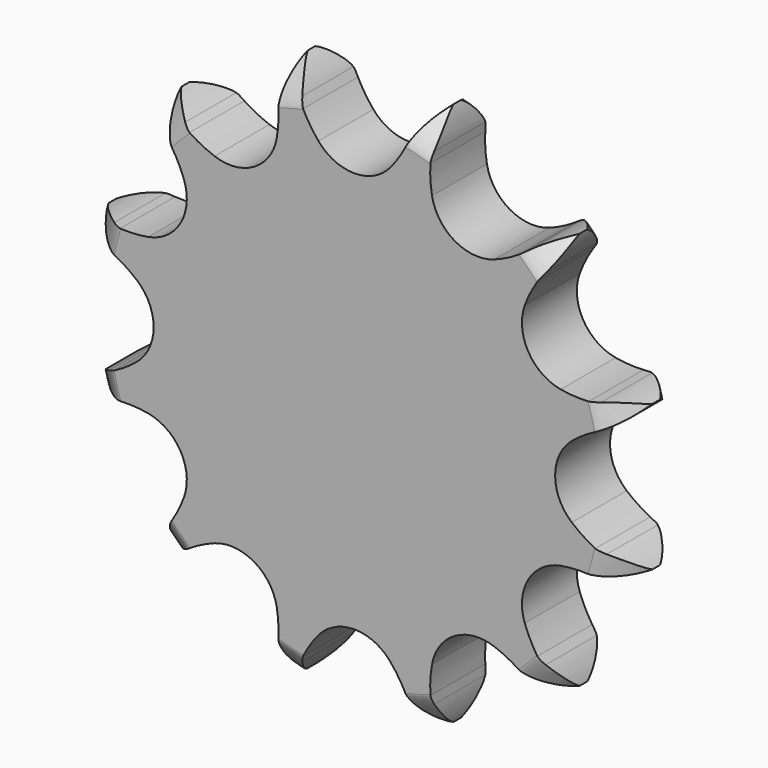
from build123d import *

# Parameters (mm, degrees)
F5_DEPTH = 5.1013001


# Not quite as in the source:
# - a fillet or chamfer that OpenCascade refuses, or shapes differently, is made with other operations: its cross-section is extruded or revolved along the edge and cut away or added


with BuildPart() as f1:
    # F0 (on Right) → F1 (revolve)
    with BuildSketch(Plane.YZ):
        Polygon((5.1003, 21), (0, 21), (0, 0), (5.1003, 0), (5.1003, 15), align=None)
    revolve(axis=Axis((0, 2.55015, 0), (0, 1, 0)))

    # F2: fillet of radius 2.75 on 1 edges, made by hand

    # F2_s1 → F2_t2 (revolve, cut)
    with BuildSketch(Plane.YZ):
        with BuildLine():
            add(Edge.make_bspline(
                [(2.75, 21), (0, 21), (0, 18.25)],
                knots=[0, 0, 0, 1, 1, 1], degree=2, weights=[1, 0.25, 1]))
            Line((0, 18.25), (0, 21))
            Line((0, 21), (2.75, 21))
        make_face()
    revolve(axis=Axis((0, 0, 0), (0, 1, 0)), mode=Mode.SUBTRACT)

    # F3: fillet of radius 2.25 on 1 edges, made by hand

    # F3_s1 → F3_t2 (revolve, cut)
    with BuildSketch(Plane.YZ):
        with BuildLine():
            add(Edge.make_bspline(
                [(2.8503, 21), (5.1003, 21), (5.1003, 18.75)],
                knots=[0, 0, 0, 1, 1, 1], degree=2, weights=[1, 0.25, 1]))
            Line((5.1003, 18.75), (5.1003, 21))
            Line((5.1003, 21), (2.8503, 21))
        make_face()
    revolve(axis=Axis((0, 5.1003, 0), (0, 1, 0)), mode=Mode.SUBTRACT)

    # F4 (on Front) → F5 (intersect, through all)
    with BuildSketch(Plane.XZ):
        with BuildLine():
            ThreePointArc((2.6688988398, 16.1610279679), (0, 14.9165), (-2.6688988398, 16.1610279679))
            ThreePointArc((-2.6688988398, 16.1610279679), (-3.2918405608, 16.997783911), (-3.8134287394, 17.9012011279))
            Line((-3.8134287394, 17.9012011279), (-4.1168666624, 18.5053956993))
            ThreePointArc((-4.1168666624, 18.5053956993), (-4.6860108551, 19.4160194738), (-5.4140261854, 20.2054207974))
            ThreePointArc((-5.4140261854, 20.2054207974), (-5.6498052939, 19.1577715323), (-5.6873867361, 18.0845761139))
            Line((-5.6873867361, 18.0845761139), (-5.6480744001, 17.4096093047))
            ThreePointArc((-5.6480744001, 17.4096093047), (-5.6480744046, 16.3664329553), (-5.7691797885, 15.3303101913))
            ThreePointArc((-5.7691797885, 15.3303101913), (-7.45825, 12.9180679356), (-10.3918481793, 12.6614113515))
            ThreePointArc((-10.3918481793, 12.6614113515), (-11.3497095063, 13.0745923945), (-12.2531267278, 13.5961805653))
            Line((-12.2531267278, 13.5961805653), (-12.8180089633, 13.9677094515))
            ThreePointArc((-12.8180089633, 13.9677094515), (-13.7662141799, 14.4717606771), (-14.791394612, 14.791394612))
            ThreePointArc((-14.791394612, 14.791394612), (-14.4717606771, 13.7662141799), (-13.9677094515, 12.8180089633))
            Line((-13.9677094515, 12.8180089633), (-13.5961805653, 12.2531267278))
            ThreePointArc((-13.5961805653, 12.2531267278), (-13.0745923945, 11.3497095063), (-12.6614113515, 10.3918481793))
            ThreePointArc((-12.6614113515, 10.3918481793), (-12.9180679356, 7.45825), (-15.3303101913, 5.7691797885))
            ThreePointArc((-15.3303101913, 5.7691797885), (-16.3664329553, 5.6480744046), (-17.4096093047, 5.6480744001))
            Line((-17.4096093047, 5.6480744001), (-18.0845761139, 5.6873867361))
            ThreePointArc((-18.0845761139, 5.6873867361), (-19.1577715323, 5.6498052939), (-20.2054207974, 5.4140261854))
            ThreePointArc((-20.2054207974, 5.4140261854), (-19.4160194738, 4.6860108551), (-18.5053956993, 4.1168666624))
            Line((-18.5053956993, 4.1168666624), (-17.9012011279, 3.8134287394))
            ThreePointArc((-17.9012011279, 3.8134287394), (-16.997783911, 3.2918405608), (-16.1610279679, 2.6688988398))
            ThreePointArc((-16.1610279679, 2.6688988398), (-14.9165, 0), (-16.1610279679, -2.6688988398))
            ThreePointArc((-16.1610279679, -2.6688988398), (-16.997783911, -3.2918405608), (-17.9012011279, -3.8134287394))
            Line((-17.9012011279, -3.8134287394), (-18.5053956993, -4.1168666624))
            ThreePointArc((-18.5053956993, -4.1168666624), (-19.4160194738, -4.6860108551), (-20.2054207974, -5.4140261854))
            ThreePointArc((-20.2054207974, -5.4140261854), (-19.1577715323, -5.6498052939), (-18.0845761139, -5.6873867361))
            Line((-18.0845761139, -5.6873867361), (-17.4096093047, -5.6480744001))
            ThreePointArc((-17.4096093047, -5.6480744001), (-16.3664329553, -5.6480744046), (-15.3303101913, -5.7691797885))
            ThreePointArc((-15.3303101913, -5.7691797885), (-12.9180679356, -7.45825), (-12.6614113515, -10.3918481793))
            ThreePointArc((-12.6614113515, -10.3918481793), (-13.0745923945, -11.3497095063), (-13.5961805653, -12.2531267278))
            Line((-13.5961805653, -12.2531267278), (-13.9677094515, -12.8180089633))
            ThreePointArc((-13.9677094515, -12.8180089633), (-14.4717606771, -13.7662141799), (-14.791394612, -14.791394612))
            ThreePointArc((-14.791394612, -14.791394612), (-13.7662141799, -14.4717606771), (-12.8180089633, -13.9677094515))
            Line((-12.8180089633, -13.9677094515), (-12.2531267278, -13.5961805653))
            ThreePointArc((-12.2531267278, -13.5961805653), (-11.3497095063, -13.0745923945), (-10.3918481793, -12.6614113515))
            ThreePointArc((-10.3918481793, -12.6614113515), (-7.45825, -12.9180679356), (-5.7691797885, -15.3303101913))
            ThreePointArc((-5.7691797885, -15.3303101913), (-5.6480744046, -16.3664329553), (-5.6480744001, -17.4096093047))
            Line((-5.6480744001, -17.4096093047), (-5.6873867361, -18.0845761139))
            ThreePointArc((-5.6873867361, -18.0845761139), (-5.6498052939, -19.1577715323), (-5.4140261854, -20.2054207974))
            ThreePointArc((-5.4140261854, -20.2054207974), (-4.6860108551, -19.4160194738), (-4.1168666624, -18.5053956993))
            Line((-4.1168666624, -18.5053956993), (-3.8134287394, -17.9012011279))
            ThreePointArc((-3.8134287394, -17.9012011279), (-3.2918405608, -16.997783911), (-2.6688988398, -16.1610279679))
            ThreePointArc((-2.6688988398, -16.1610279679), (0, -14.9165), (2.6688988398, -16.1610279679))
            ThreePointArc((2.6688988398, -16.1610279679), (3.2918405608, -16.997783911), (3.8134287394, -17.9012011279))
            Line((3.8134287394, -17.9012011279), (4.1168666624, -18.5053956993))
            ThreePointArc((4.1168666624, -18.5053956993), (4.6860108551, -19.4160194738), (5.4140261854, -20.2054207974))
            ThreePointArc((5.4140261854, -20.2054207974), (5.6498052939, -19.1577715323), (5.6873867361, -18.0845761139))
            Line((5.6873867361, -18.0845761139), (5.6480744001, -17.4096093047))
            ThreePointArc((5.6480744001, -17.4096093047), (5.6480744046, -16.3664329553), (5.7691797885, -15.3303101913))
            ThreePointArc((5.7691797885, -15.3303101913), (7.45825, -12.9180679356), (10.3918481793, -12.6614113515))
            ThreePointArc((10.3918481793, -12.6614113515), (11.3497095063, -13.0745923945), (12.2531267278, -13.5961805653))
            Line((12.2531267278, -13.5961805653), (12.8180089633, -13.9677094515))
            ThreePointArc((12.8180089633, -13.9677094515), (13.7662141799, -14.4717606771), (14.791394612, -14.791394612))
            ThreePointArc((14.791394612, -14.791394612), (14.4717606771, -13.7662141799), (13.9677094515, -12.8180089633))
            Line((13.9677094515, -12.8180089633), (13.5961805653, -12.2531267278))
            ThreePointArc((13.5961805653, -12.2531267278), (13.0745923945, -11.3497095063), (12.6614113515, -10.3918481793))
            ThreePointArc((12.6614113515, -10.3918481793), (12.9180679356, -7.45825), (15.3303101913, -5.7691797885))
            ThreePointArc((15.3303101913, -5.7691797885), (16.3664329553, -5.6480744046), (17.4096093047, -5.6480744001))
            Line((17.4096093047, -5.6480744001), (18.0845761139, -5.6873867361))
            ThreePointArc((18.0845761139, -5.6873867361), (19.1577715323, -5.6498052939), (20.2054207974, -5.4140261854))
            ThreePointArc((20.2054207974, -5.4140261854), (19.4160194738, -4.6860108551), (18.5053956993, -4.1168666624))
            Line((18.5053956993, -4.1168666624), (17.9012011279, -3.8134287394))
            ThreePointArc((17.9012011279, -3.8134287394), (16.997783911, -3.2918405608), (16.1610279679, -2.6688988398))
            ThreePointArc((16.1610279679, -2.6688988398), (14.9165, 0), (16.1610279679, 2.6688988398))
            ThreePointArc((16.1610279679, 2.6688988398), (16.997783911, 3.2918405608), (17.9012011279, 3.8134287394))
            Line((17.9012011279, 3.8134287394), (18.5053956993, 4.1168666624))
            ThreePointArc((18.5053956993, 4.1168666624), (19.4160194738, 4.6860108551), (20.2054207974, 5.4140261854))
            ThreePointArc((20.2054207974, 5.4140261854), (19.1577715323, 5.6498052939), (18.0845761139, 5.6873867361))
            Line((18.0845761139, 5.6873867361), (17.4096093047, 5.6480744001))
            ThreePointArc((17.4096093047, 5.6480744001), (16.3664329553, 5.6480744046), (15.3303101913, 5.7691797885))
            ThreePointArc((15.3303101913, 5.7691797885), (12.9180679356, 7.45825), (12.6614113515, 10.3918481793))
            ThreePointArc((12.6614113515, 10.3918481793), (13.0745923945, 11.3497095063), (13.5961805653, 12.2531267278))
            Line((13.5961805653, 12.2531267278), (13.9677094515, 12.8180089633))
            ThreePointArc((13.9677094515, 12.8180089633), (14.4717606771, 13.7662141799), (14.791394612, 14.791394612))
            ThreePointArc((14.791394612, 14.791394612), (13.7662141799, 14.4717606771), (12.8180089633, 13.9677094515))
            Line((12.8180089633, 13.9677094515), (12.2531267278, 13.5961805653))
            ThreePointArc((12.2531267278, 13.5961805653), (11.3497095063, 13.0745923945), (10.3918481793, 12.6614113515))
            ThreePointArc((10.3918481793, 12.6614113515), (7.45825, 12.9180679356), (5.7691797885, 15.3303101913))
            ThreePointArc((5.7691797885, 15.3303101913), (5.6480744046, 16.3664329553), (5.6480744001, 17.4096093047))
            Line((5.6480744001, 17.4096093047), (5.6873867361, 18.0845761139))
            ThreePointArc((5.6873867361, 18.0845761139), (5.6498052939, 19.1577715323), (5.4140261854, 20.2054207974))
            ThreePointArc((5.4140261854, 20.2054207974), (4.6860108551, 19.4160194738), (4.1168666624, 18.5053956993))
            Line((4.1168666624, 18.5053956993), (3.8134287394, 17.9012011279))
            ThreePointArc((3.8134287394, 17.9012011279), (3.2918405608, 16.997783911), (2.6688988398, 16.1610279679))
        make_face()
    extrude(amount=-F5_DEPTH, mode=Mode.INTERSECT)


solid = f1.part
